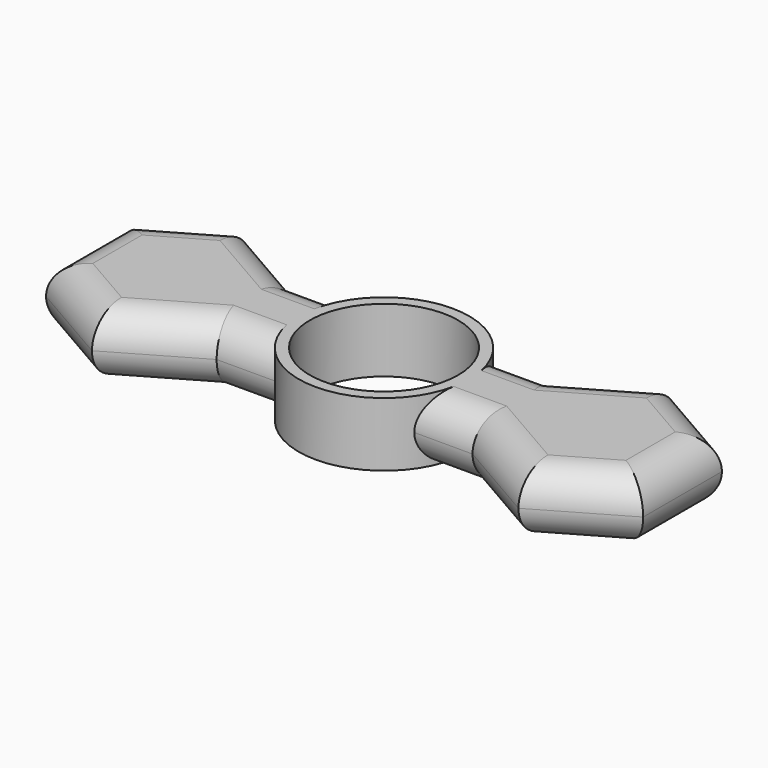
from build123d import *

# Parameters (mm, degrees)
F0_R     = 12.7
F0_R_2   = 11.049
F1_DEPTH = 4.7625
F3_DEPTH = 4.7625
F4_R     = 4.76249
F5_R     = 4.76249


# Not quite as in the source:
# - a fillet or chamfer is up to 0.001 mm smaller than in the source, because OpenCascade refuses the exact size


with BuildPart() as f1:
    # F0 (on Top) → F1 (new body, symmetric)
    with BuildSketch(Plane.XY):
        Circle(F0_R)
        Circle(F0_R_2, mode=Mode.SUBTRACT)
    extrude(amount=F1_DEPTH, both=True)

    # F2 (on Top) → F3 (join, symmetric)
    with BuildSketch(Plane.XY):
        with BuildLine():
            ThreePointArc((-10.3695065778, -7.3323484187), (-12.7, 0), (-10.3695065778, 7.3323484187))
            Line((-10.3695065778, 7.3323484187), (-19.05, 7.3323484187))
            Line((-19.05, 7.3323484187), (-31.75, 14.6646968374))
            Line((-31.75, 14.6646968374), (-44.45, 7.3323484187))
            Line((-44.45, 7.3323484187), (-44.45, -7.3323484187))
            Line((-44.45, -7.3323484187), (-31.75, -14.6646968374))
            Line((-31.75, -14.6646968374), (-19.05, -7.3323484187))
            Line((-19.05, -7.3323484187), (-10.3695065778, -7.3323484187))
        make_face()
        with BuildLine():
            Line((44.45, -7.3323484187), (44.45, 7.3323484187))
            Line((44.45, 7.3323484187), (31.75, 14.6646968374))
            Line((31.75, 14.6646968374), (19.05, 7.3323484187))
            Line((19.05, 7.3323484187), (10.3695065778, 7.3323484187))
            ThreePointArc((10.3695065778, 7.3323484187), (12.7, 0), (10.3695065778, -7.3323484187))
            Line((10.3695065778, -7.3323484187), (19.05, -7.3323484187))
            Line((19.05, -7.3323484187), (31.75, -14.6646968374))
            Line((31.75, -14.6646968374), (44.45, -7.3323484187))
        make_face()
    extrude(amount=F3_DEPTH, both=True)

    # F4 (radius 4.7625 in the source; OpenCascade refuses exactly that, so slightly less here)
    f4_edges = [f1.edges().sort_by_distance(p)[0] for p in [
        (38.1, -10.998523, 4.7625),
        (44.45, 0, 4.7625),
        (25.4, -10.998523, 4.7625),
        (14.709753, -7.332348, 4.7625),
        (14.709753, 7.332348, 4.7625),
        (25.4, 10.998523, 4.7625),
        (38.1, 10.998523, 4.7625),
        (14.709753, -7.332348, -4.7625),
        (25.4, -10.998523, -4.7625),
        (38.1, -10.998523, -4.7625),
        (44.45, 0, -4.7625),
        (14.709753, 7.332348, -4.7625),
        (25.4, 10.998523, -4.7625),
        (38.1, 10.998523, -4.7625),
    ]]
    fillet(f4_edges, radius=F4_R)

    # F5 (radius 4.7625 in the source; OpenCascade refuses exactly that, so slightly less here)
    f5_edges = [f1.edges().sort_by_distance(p)[0] for p in [
        (-38.1, 10.998523, 4.7625),
        (-25.4, 10.998523, 4.7625),
        (-14.709753, 7.332348, 4.7625),
        (-14.709753, -7.332348, 4.7625),
        (-25.4, -10.998523, 4.7625),
        (-38.1, -10.998523, 4.7625),
        (-44.45, 0, -4.7625),
        (-44.45, 0, 4.7625),
        (-25.4, -10.998523, -4.7625),
        (-38.1, -10.998523, -4.7625),
        (-14.709753, -7.332348, -4.7625),
        (-14.709753, 7.332348, -4.7625),
        (-25.4, 10.998523, -4.7625),
        (-38.1, 10.998523, -4.7625),
    ]]
    fillet(f5_edges, radius=F5_R)


solid = f1.part
